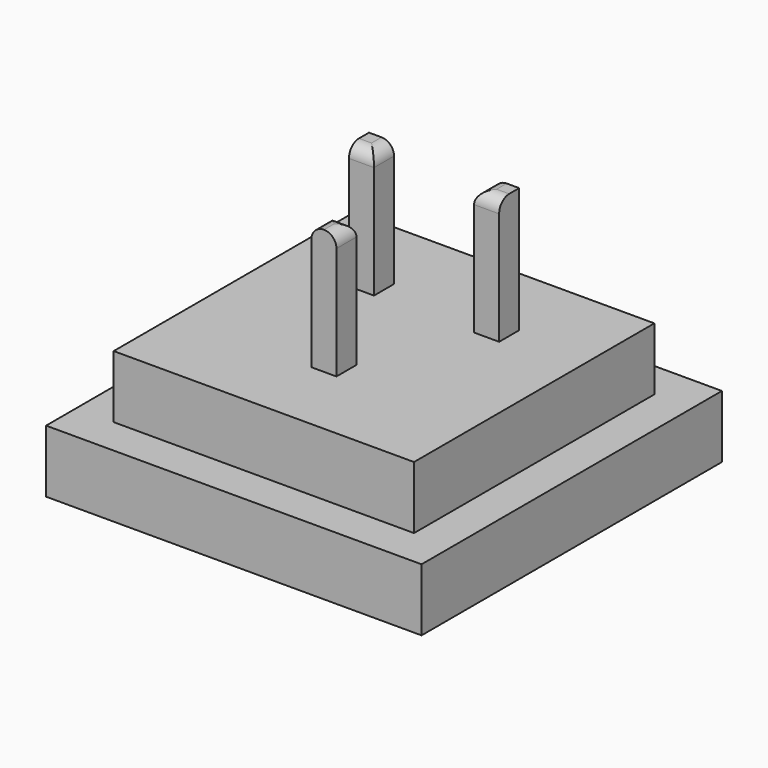
from build123d import *

# Parameters (mm, degrees)
F0_W     = 150
F0_H     = 150
F1_DEPTH = 25
F2_W     = 120
F2_H     = 120
F3_DEPTH = 25
F4_W     = 10
F4_H     = 10
F5_DEPTH = 50
F6_R     = 4.99999


# Not quite as in the source:
# - a fillet or chamfer is up to 0.001 mm smaller than in the source, because OpenCascade refuses the exact size


with BuildPart() as f1:
    # F0 (on Top) → F1 (new body)
    with BuildSketch(Plane.XY):
        Rectangle(F0_W, F0_H)
    extrude(amount=F1_DEPTH)

    # F2 (on face) → F3 (join)
    with BuildSketch(Plane.XY.offset(25)):
        Rectangle(F2_W, F2_H)
    extrude(amount=F3_DEPTH)

    # F4 (on face) → F5 (join)
    with BuildSketch(Plane.XY.offset(50)):
        with Locations((0, -25)):
            Rectangle(F4_W, F4_H)
        with Locations((-25, 25)):
            Rectangle(F4_W, F4_H)
        with Locations((25, 25)):
            Rectangle(F4_W, F4_H)
    extrude(amount=F5_DEPTH)

    # F6 (radius 5 in the source; OpenCascade refuses exactly that, so slightly less here)
    f6_edges = [f1.edges().sort_by_distance(p)[0] for p in [
        (-25, 20, 100),
        (-20, 25, 100),
        (25, 20, 100),
        (20, 25, 100),
        (-5, -25, 100),
        (0, -20, 100),
        (5, -25, 100),
    ]]
    fillet(f6_edges, radius=F6_R)


solid = f1.part
